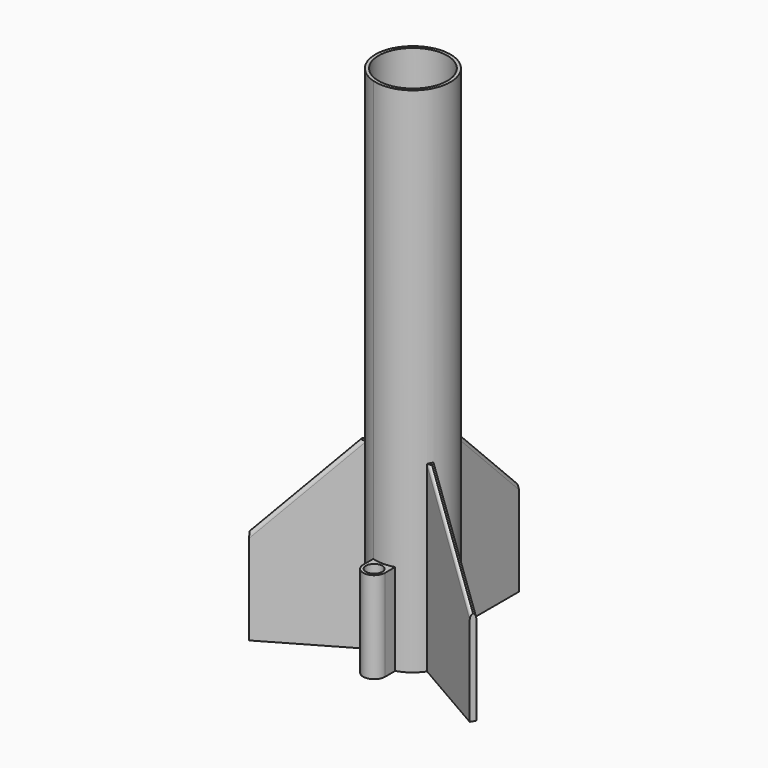
from build123d import *

# Parameters (mm, degrees)
F0_R         = 9.375
F1_DEPTH     = 140
F2_DEPTH     = 50
F3_SIZE      = 24
F4_T4_DEPTH  = 38.941125497
F4_T10_DEPTH = 38.941125497
F5_COUNT     = 3
F0_R_2       = 2.25
F6_DEPTH     = 10
F7_START     = 69.5
F0_R_3       = 7.5
F7_DEPTH     = 2.5
F8_DEPTH     = 25
F9_R         = 2
F10_DEPTH    = 25


# Not quite as in the source:
# - a fillet or chamfer that OpenCascade refuses, or shapes differently, is made with other operations: its cross-section is extruded or revolved along the edge and cut away or added


with BuildPart() as f1:
    # F0 (on Top) → F1 (new body)
    with BuildSketch(Plane.XY):
        with BuildLine():
            ThreePointArc((3, -9.801147892), (8.2405248619, -6.0955926701), (10.25, 0))
            ThreePointArc((10.25, 0), (7.5083287088, 6.9776428685), (0.75, 10.2225241501))
            ThreePointArc((0.75, 10.2225241501), (0, 10.25), (-0.75, 10.2225241501))
            ThreePointArc((-0.75, 10.2225241501), (-10.185896402, 1.1445586432), (-3, -9.801147892))
            ThreePointArc((-3, -9.801147892), (-1.5166961062, -10.1371659216), (-1.65e-08, -10.25))
            ThreePointArc((-1.65e-08, -10.25), (1.5166960899, -10.137165924), (3, -9.801147892))
        make_face()
        Circle(F0_R, mode=Mode.SUBTRACT)
    extrude(amount=F1_DEPTH)

    # F0 (on Top) → F2 (join)
    with BuildSketch(Plane.XY):
        with BuildLine():
            ThreePointArc((-0.75, 10.2225241501), (0, 10.25), (0.75, 10.2225241501))
            Line((0.75, 10.2225241501), (0.75, 35.2225241501))
            Line((0.75, 35.2225241501), (-0.75, 35.2225241501))
            Line((-0.75, 35.2225241501), (-0.75, 10.2225241501))
        make_face()
    extrude(amount=F2_DEPTH)

    # F3
    f3_edges = [f1.edges().sort_by_distance(p)[0] for p in [
        (0, 35.222524, 50),
    ]]
    chamfer(f3_edges, length=F3_SIZE)

    # F4: fillet of radius 1 on 2 edges, made by hand


with BuildPart() as f4_tool2:
    # F4_s3 → F4_t4 (new body)
    with BuildSketch(Plane(origin=(0, -21.1565048779, 21.1565048779), x_dir=(1, 0, 0), z_dir=(0, 0.7071067812, -0.7071067812))):
        with BuildLine():
            ThreePointArc((0.75, -42.2908619879), (0.4571067812, -42.9979687691), (-0.25, -43.2908619879))
            Line((-0.25, -43.2908619879), (-0.25, -43.3108619879))
            Line((-0.25, -43.3108619879), (0.77, -43.3108619879))
            Line((0.77, -43.3108619879), (0.77, -42.2908619879))
            Line((0.77, -42.2908619879), (0.75, -42.2908619879))
        make_face()
    extrude(amount=F4_T4_DEPTH)

    split(bisect_by=Plane.XZ.offset(-35.2225241501), keep=Keep.TOP)

    split(bisect_by=Plane.XY.offset(50), keep=Keep.BOTTOM)


with BuildPart() as f1_1:
    add(f1.part)

    # F4_t1: cut F4_tool2
    add(f4_tool2.part, mode=Mode.SUBTRACT)


with BuildPart() as f4_tool8:
    # F4_s9 → F4_t10 (new body)
    with BuildSketch(Plane(origin=(0, -21.1565048779, 21.1565048779), x_dir=(1, 0, 0), z_dir=(0, 0.7071067812, -0.7071067812))):
        with BuildLine():
            ThreePointArc((0.25, -43.2908619879), (-0.4571067812, -42.9979687691), (-0.75, -42.2908619879))
            Line((-0.75, -42.2908619879), (-0.77, -42.2908619879))
            Line((-0.77, -42.2908619879), (-0.77, -43.3108619879))
            Line((-0.77, -43.3108619879), (0.25, -43.3108619879))
            Line((0.25, -43.3108619879), (0.25, -43.2908619879))
        make_face()
    extrude(amount=F4_T10_DEPTH)

    split(bisect_by=Plane.XZ.offset(-35.2225241501), keep=Keep.TOP)

    split(bisect_by=Plane.XY.offset(50), keep=Keep.BOTTOM)


with BuildPart() as f1_2:
    add(f1_1.part)

    # F4_t7: cut F4_tool8
    add(f4_tool8.part, mode=Mode.SUBTRACT)


with BuildPart() as f5_1:
    # F5: instance of F1
    add(f1_2.part.rotate(Axis((0, 0, 0), (0, 0, -1)), 1 * 360 / F5_COUNT))


with BuildPart() as f5_2:
    # F5: instance of F1
    add(f1_2.part.rotate(Axis((0, 0, 0), (0, 0, -1)), 2 * 360 / F5_COUNT))


with BuildPart() as f1_3:
    add(f1_2.part)

    add(f5_1.part)  # F6 merges F5_1

    add(f5_2.part)  # F6 merges F5_2
    # F0 (on Top) → F6 (join)
    with BuildSketch(Plane.XY):
        with BuildLine():
            ThreePointArc((3, -13.25), (2.1213203377, -11.1286796506), (-1.65e-08, -10.25))
            ThreePointArc((-1.65e-08, -10.25), (-2.1213203494, -11.1286796623), (-3, -13.25))
            ThreePointArc((-3, -13.25), (0, -16.25), (3, -13.25))
        make_face()
        with Locations((0, -13.25)):
            Circle(F0_R_2, mode=Mode.SUBTRACT)
        with BuildLine():
            ThreePointArc((-3, -13.25), (-2.1213203494, -11.1286796623), (-1.65e-08, -10.25))
            ThreePointArc((-1.65e-08, -10.25), (-1.5166961062, -10.1371659216), (-3, -9.801147892))
            Line((-3, -9.801147892), (-3, -13.25))
        make_face()
        with BuildLine():
            Line((3, -13.25), (3, -9.801147892))
            ThreePointArc((3, -9.801147892), (1.5166960899, -10.137165924), (-1.65e-08, -10.25))
            ThreePointArc((-1.65e-08, -10.25), (2.1213203377, -11.1286796506), (3, -13.25))
        make_face()
    extrude(amount=F6_DEPTH)

    # F0 (on Top) → F7 (join)
    with BuildSketch(Plane.XY.offset(F7_START)):
        Circle(F0_R)
        Circle(F0_R_3, mode=Mode.SUBTRACT)
    extrude(amount=F7_DEPTH)

    # F0 (on Top) → F8 (join)
    with BuildSketch(Plane.XY):
        with BuildLine():
            ThreePointArc((3, -13.25), (2.1213203377, -11.1286796506), (-1.65e-08, -10.25))
            ThreePointArc((-1.65e-08, -10.25), (-2.1213203494, -11.1286796623), (-3, -13.25))
            ThreePointArc((-3, -13.25), (0, -16.25), (3, -13.25))
        make_face()
        with Locations((0, -13.25)):
            Circle(F0_R_2, mode=Mode.SUBTRACT)
        with BuildLine():
            Line((3, -13.25), (3, -9.801147892))
            ThreePointArc((3, -9.801147892), (1.5166960899, -10.137165924), (-1.65e-08, -10.25))
            ThreePointArc((-1.65e-08, -10.25), (2.1213203377, -11.1286796506), (3, -13.25))
        make_face()
        with BuildLine():
            ThreePointArc((-3, -13.25), (-2.1213203494, -11.1286796623), (-1.65e-08, -10.25))
            ThreePointArc((-1.65e-08, -10.25), (-1.5166961062, -10.1371659216), (-3, -9.801147892))
            Line((-3, -9.801147892), (-3, -13.25))
        make_face()
    extrude(amount=F8_DEPTH)

    # F9 (on Right) → F10 (cut)
    with BuildSketch(Plane.YZ):
        with Locations((0, 112.2226320051)):
            Circle(F9_R)
        with Locations((0, 101.8494740129)):
            Circle(F9_R)
    extrude(amount=-F10_DEPTH, mode=Mode.SUBTRACT)


solid = f1_3.part
